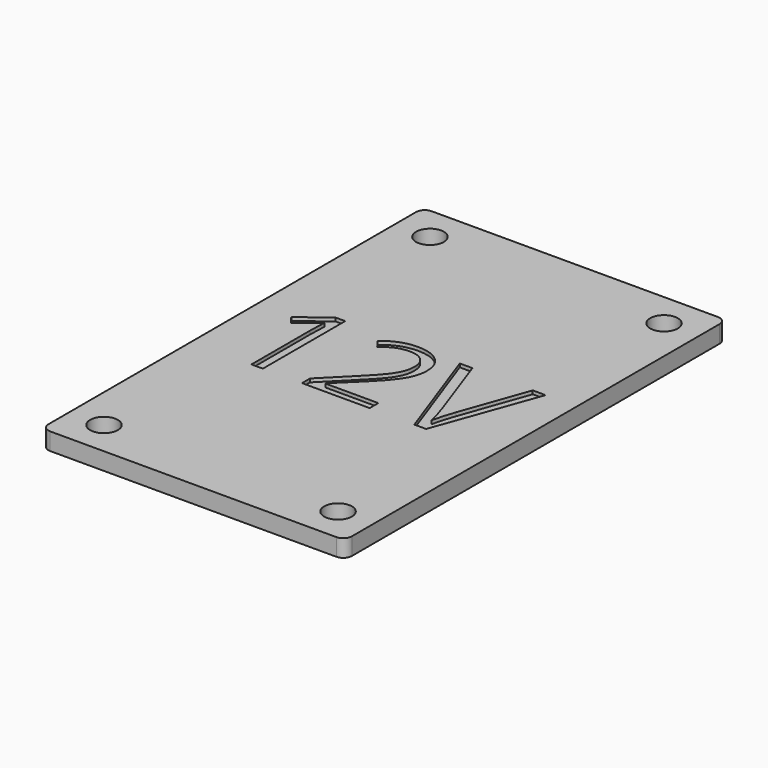
from build123d import *

# Parameters (mm, degrees)
F0_W          = 35
F0_H          = 55
F0_R          = 1.6
F1_DEPTH      = 2
F2_DEPTH      = 3
F3_R          = 1
F4_W          = 20
F4_H          = 4
F5_DEPTH      = 5
F6_TEXT_SIZE  = 16.6348986311
F7_DEPTH      = 0.4
F7_DEPTH_BACK = 25


# Not quite as in the source:
# - Text() gives the source's letters only with a copy of the font that has no kerning and outlines rounded to 1/6400 em; it was checked with that copy


with BuildPart() as f1:
    # F0 (on Top) → F1 (new body)
    with BuildSketch(Plane.XY):
        Rectangle(F0_W, F0_H)
        with Locations((-13.5, -23.5)):
            Circle(F0_R, mode=Mode.SUBTRACT)
        with Locations((13.5, -23.5)):
            Circle(F0_R, mode=Mode.SUBTRACT)
        with Locations((-13.5, 23.5)):
            Circle(F0_R, mode=Mode.SUBTRACT)
        with BuildLine():
            ThreePointArc((14.9, -18.7), (10.5159379566, -20.5159379566), (8.7, -24.9))
            Line((8.7, -24.9), (-8.7, -24.9))
            ThreePointArc((-8.7, -24.9), (-10.5159379566, -20.5159379566), (-14.9, -18.7))
            Line((-14.9, -18.7), (-14.9, 18.7))
            ThreePointArc((-14.9, 18.7), (-10.5159379566, 20.5159379566), (-8.7, 24.9))
            Line((-8.7, 24.9), (8.7, 24.9))
            ThreePointArc((8.7, 24.9), (10.5159379566, 20.5159379566), (14.9, 18.7))
            Line((14.9, 18.7), (14.9, -18.7))
        make_face(mode=Mode.SUBTRACT)
        with Locations((13.5, 23.5)):
            Circle(F0_R, mode=Mode.SUBTRACT)
    extrude(amount=-F1_DEPTH)

    # F0 (on Top) → F2 (join)
    with BuildSketch(Plane.XY):
        with BuildLine():
            Line((-8.7, -24.9), (8.7, -24.9))
            ThreePointArc((8.7, -24.9), (10.5159379566, -20.5159379566), (14.9, -18.7))
            Line((14.9, -18.7), (14.9, 18.7))
            ThreePointArc((14.9, 18.7), (10.5159379566, 20.5159379566), (8.7, 24.9))
            Line((8.7, 24.9), (-8.7, 24.9))
            ThreePointArc((-8.7, 24.9), (-10.5159379566, 20.5159379566), (-14.9, 18.7))
            Line((-14.9, 18.7), (-14.9, -18.7))
            ThreePointArc((-14.9, -18.7), (-10.5159379566, -20.5159379566), (-8.7, -24.9))
        make_face()
    extrude(amount=-F2_DEPTH)

    # F3
    f3_edges = [f1.edges().sort_by_distance(p)[0] for p in [
        (17.5, 27.5, -1),
        (-17.5, 27.5, -1),
        (17.5, -27.5, -1),
        (-17.5, -27.5, -1),
    ]]
    fillet(f3_edges, radius=F3_R)

    # F4 (on Top) → F5 (join)
    with BuildSketch(Plane.XY):
        with Locations((0, -10)):
            Rectangle(F4_W, F4_H)
    extrude(amount=-F5_DEPTH)

    # F6 (on Top) → F7 (cut, two sides)
    with BuildSketch(Plane.XY) as f7_sk:
        with Locations((-15, -5.9771270144)):
            Text('12V', F6_TEXT_SIZE, font='Open Sans', text_align=(TextAlign.LEFT, TextAlign.BOTTOM))
    extrude(amount=-F7_DEPTH, mode=Mode.SUBTRACT)
    extrude(f7_sk.sketch, amount=F7_DEPTH_BACK, mode=Mode.SUBTRACT)


solid = f1.part
